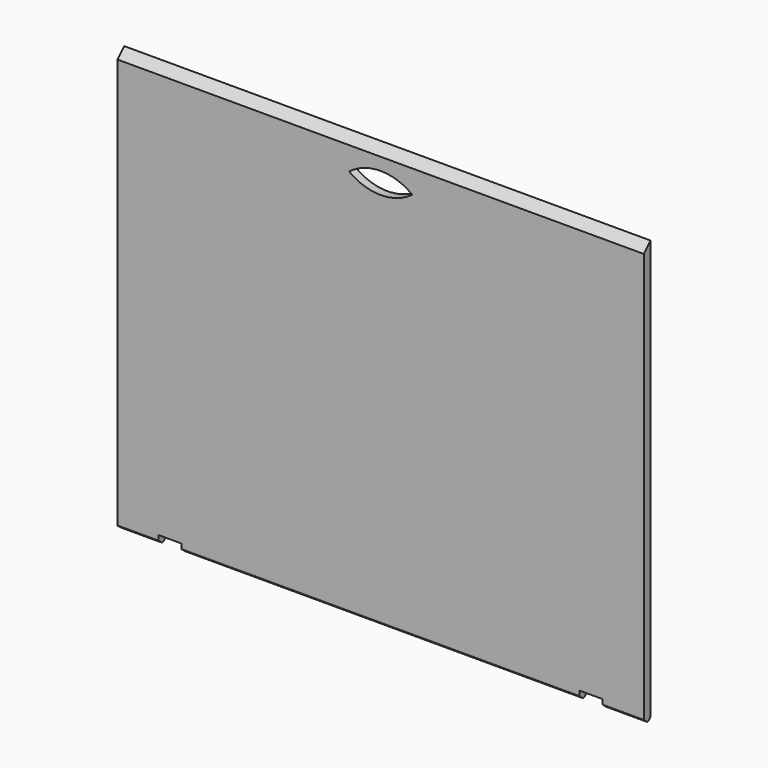
from build123d import *

# Parameters (mm, degrees)
F0_W     = 250
F0_H     = 197
F1_DEPTH = 4
F3_W     = 11
F3_H     = 4
F4_DEPTH = 0.5
F5_DEPTH = 250
F6_DEPTH = 25
F8_DEPTH = 25
F9_SIZE  = 3.99999


# Not quite as in the source:
# - a fillet or chamfer is up to 0.001 mm smaller than in the source, because OpenCascade refuses the exact size


with BuildPart() as f1:
    # F0 (on Front) → F1 (new body)
    with BuildSketch(Plane.XZ):
        Rectangle(F0_W, F0_H)
    extrude(amount=F1_DEPTH)

    # F3 (on face) → F4 (cut)
    with BuildSketch(Plane(origin=(0, 0, -98.5), x_dir=(1, 0, 0), z_dir=(0, 0, -1))):
        Polygon((-105.5, 0), (-94.5, 0), (-94.5, 4), (-105.5, 4), (-105.5, 2), align=None)
        with Locations((100, 2)):
            Rectangle(F3_W, F3_H)
    extrude(amount=-F4_DEPTH, mode=Mode.SUBTRACT)

    # F2 (on face) → F5 (join)
    with BuildSketch(Plane.YZ.offset(125)):
        with BuildLine():
            Line((-3.3228756555, -98.5), (-4, -98.5))
            Line((-4, -98.5), (-4, -100))
            ThreePointArc((-4, -100), (-3.8228756555, -99.1771243445), (-3.3228756555, -98.5))
        make_face()
        with BuildLine():
            ThreePointArc((-3.3228756555, -98.5), (-3.8228756555, -99.1771243445), (-4, -100))
            Line((-4, -100), (0, -100))
            ThreePointArc((0, -100), (-0.1771243445, -99.1771243445), (-0.6771243445, -98.5))
            Line((-0.6771243445, -98.5), (-3.3228756555, -98.5))
        make_face()
        with BuildLine():
            ThreePointArc((-0.6771243445, -98.5), (-0.1771243445, -99.1771243445), (0, -100))
            Line((0, -100), (0, -98.5))
            Line((0, -98.5), (-0.6771243445, -98.5))
        make_face()
        with BuildLine():
            Line((0, -100), (-4, -100))
            ThreePointArc((-4, -100), (-3.9878535848, -100.2200866318), (-3.9515618745, -100.4375))
            Line((-3.9515618745, -100.4375), (-2, -102))
            ThreePointArc((-2, -102), (-0.5857864376, -101.4142135624), (0, -100))
        make_face()
    extrude(amount=-F5_DEPTH)

    # F3 (on face) → F6 (cut)
    with BuildSketch(Plane(origin=(0, 0, -98.5), x_dir=(1, 0, 0), z_dir=(0, 0, -1))):
        Polygon((-105.5, 0), (-94.5, 0), (-94.5, 4), (-105.5, 4), (-105.5, 2), align=None)
        with Locations((100, 2)):
            Rectangle(F3_W, F3_H)
    extrude(amount=F6_DEPTH, mode=Mode.SUBTRACT)

    # F7 (on face) → F8 (cut)
    with BuildSketch(Plane.XZ.offset(4)):
        with BuildLine():
            ThreePointArc((-15, 83.5), (0, 78.4776194071), (15, 83.5))
            Line((15, 83.5), (5, 83.5))
            ThreePointArc((5, 83.5), (0, 78.5), (-5, 83.5))
            Line((-5, 83.5), (-15, 83.5))
        make_face()
        with BuildLine():
            Line((5, 83.5), (0, 83.5))
            Line((0, 83.5), (-5, 83.5))
            ThreePointArc((-5, 83.5), (0, 78.5), (5, 83.5))
        make_face()
        with BuildLine():
            Line((0, 83.5), (0, 88.5))
            ThreePointArc((0, 88.5), (-3.5355339059, 87.0355339059), (-5, 83.5))
            Line((-5, 83.5), (0, 83.5))
        make_face()
        with BuildLine():
            Line((0, 88.5), (0, 88.5776101571))
            ThreePointArc((0, 88.5776101571), (-7.918050974, 87.2737885484), (-15, 83.5))
            Line((-15, 83.5), (-5, 83.5))
            ThreePointArc((-5, 83.5), (-3.5355339059, 87.0355339059), (0, 88.5))
        make_face()
        with BuildLine():
            ThreePointArc((5, 83.5), (3.5355339059, 87.0355339059), (0, 88.5))
            Line((0, 88.5), (0, 83.5))
            Line((0, 83.5), (5, 83.5))
        make_face()
        with BuildLine():
            ThreePointArc((15, 83.5), (7.918050974, 87.2737885484), (0, 88.5776101571))
            Line((0, 88.5776101571), (0, 88.5))
            ThreePointArc((0, 88.5), (3.5355339059, 87.0355339059), (5, 83.5))
            Line((5, 83.5), (15, 83.5))
        make_face()
    extrude(amount=-F8_DEPTH, mode=Mode.SUBTRACT)

    # F9 (size 4 in the source; OpenCascade refuses exactly that, so slightly less here)
    f9_edges = [f1.edges().sort_by_distance(p)[0] for p in [
        (0, -4, 98.5),
    ]]
    chamfer(f9_edges, length=F9_SIZE)


solid = f1.part
